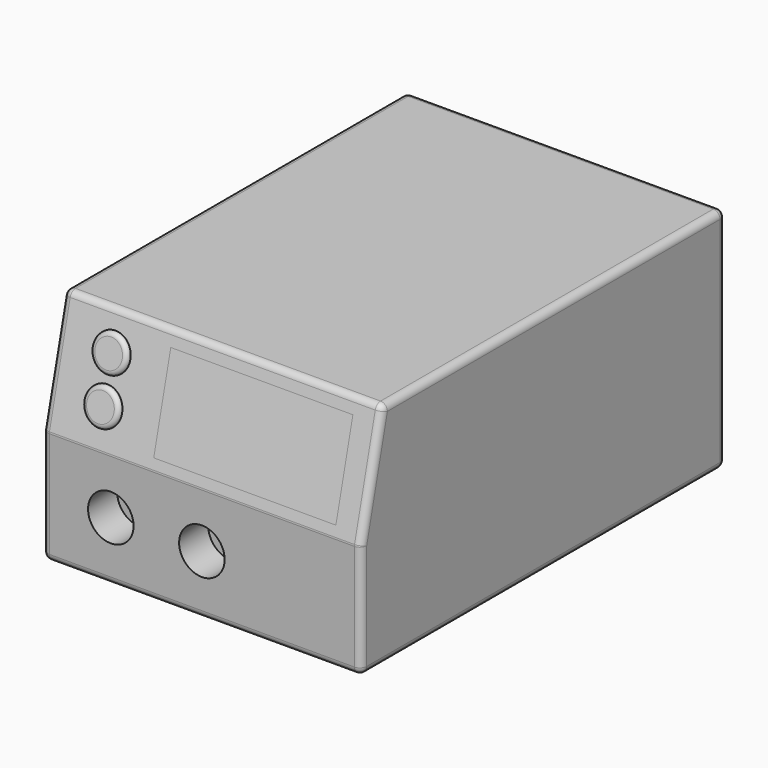
from build123d import *

# Parameters (mm, degrees)
F0_W      = 350
F0_H      = 500
F1_DEPTH  = 250
F3_DEPTH  = 350
F4_R      = 20
F5_DEPTH  = 5
F6_R      = 4.99999
F7_R      = 20
F8_DEPTH  = 5
F9_R      = 4.99999
F10_W     = 200
F10_H     = 100
F11_DEPTH = 5
F12_W     = 200
F12_H     = 100
F13_DEPTH = 5
F14_R     = 25
F15_DEPTH = 40
F16_R     = 7.5
F17_DEPTH = 60
F18_R     = 25
F19_DEPTH = 40
F20_R     = 7.5
F21_DEPTH = 60
F22_R     = 7.5
F23_R     = 12.5
F24_DEPTH = 30
F25_R     = 3
F26_DEPTH = 25
F27_W     = 55
F27_H     = 10
F28_DEPTH = 15


# Not quite as in the source:
# - a fillet or chamfer is up to 0.001 mm smaller than in the source, because OpenCascade refuses the exact size


with BuildPart() as f1:
    # F0 (on Top) → F1 (new body)
    with BuildSketch(Plane.XY):
        Rectangle(F0_W, F0_H)
    extrude(amount=F1_DEPTH)

    # F2 (on face) → F3 (cut)
    with BuildSketch(Plane.YZ.offset(175)):
        Polygon((-220, 250), (-250, 250), (-250, 125), align=None)
    extrude(amount=-F3_DEPTH, mode=Mode.SUBTRACT)

    # F10 (on face) → F11 (cut)
    with BuildSketch(Plane(origin=(0, -264.7503782148, 63.5400907716), x_dir=(1, 0, 0), z_dir=(0, -0.972387302, 0.2333729525))):
        with Locations((45, 124.7547759506)):
            Rectangle(F10_W, F10_H)
    extrude(amount=-F11_DEPTH, mode=Mode.SUBTRACT)

    # F14 (on face) → F15 (cut)
    with BuildSketch(Plane.XZ.offset(250)):
        with Locations((0, 65)):
            Circle(F14_R)
    extrude(amount=-F15_DEPTH, mode=Mode.SUBTRACT)

    # F16 (on face) → F17 (cut)
    with BuildSketch(Plane.XZ.offset(210)):
        with Locations((0, 65)):
            Circle(F16_R)
    extrude(amount=-F17_DEPTH, mode=Mode.SUBTRACT)

    # F18 (on face) → F19 (cut)
    with BuildSketch(Plane.XZ.offset(250)):
        with Locations((-100, 65)):
            Circle(F18_R)
    extrude(amount=-F19_DEPTH, mode=Mode.SUBTRACT)

    # F20 (on face) → F21 (cut)
    with BuildSketch(Plane.XZ.offset(210)):
        with Locations((-100, 65)):
            Circle(F20_R)
    extrude(amount=-F21_DEPTH, mode=Mode.SUBTRACT)

    # F22
    f22_edges = [f1.edges().sort_by_distance(p)[0] for p in [
        (175, -235, 187.5),
        (175, -250, 62.5),
        (0, -250, 125),
        (175, 15, 250),
        (175, 250, 125),
        (175, 0, 0),
        (0, -250, 0),
        (-175, -250, 62.5),
        (-175, -235, 187.5),
        (-175, 15, 250),
        (-175, 250, 125),
        (-175, 0, 0),
        (0, 250, 0),
        (0, 250, 250),
        (0, -220, 250),
    ]]
    fillet(f22_edges, radius=F22_R)

    # F23 (on face) → F24 (cut)
    with BuildSketch(Plane(origin=(0, 250, 0), x_dir=(-1, 0, 0), z_dir=(0, 1, 0))):
        with Locations((-132.5, 37.5)):
            Circle(F23_R)
    extrude(amount=-F24_DEPTH, mode=Mode.SUBTRACT)

    # F27 (on face) → F28 (cut)
    with BuildSketch(Plane(origin=(0, 250, 0), x_dir=(-1, 0, 0), z_dir=(0, 1, 0))):
        with Locations((-67.5, 37.5)):
            Rectangle(F27_W, F27_H)
    extrude(amount=-F28_DEPTH, mode=Mode.SUBTRACT)


with BuildPart() as f5:
    # F4 (on face) → F5 (new body)
    with BuildSketch(Plane(origin=(0, -264.7503782148, 63.5400907716), x_dir=(1, 0, 0), z_dir=(0, -0.972387302, 0.2333729525))):
        with Locations((-115, 151.7547759506)):
            Circle(F4_R)
    extrude(amount=F5_DEPTH)

    # F6 (radius 5 in the source; OpenCascade refuses exactly that, so slightly less here)
    f6_edges = [f5.edges().sort_by_distance(p)[0] for p in [
        (-135, -234.196855, 212.271373),
    ]]
    fillet(f6_edges, radius=F6_R)


with BuildPart() as f8:
    # F7 (on face) → F8 (new body)
    with BuildSketch(Plane(origin=(0, -264.7503782148, 63.5400907716), x_dir=(1, 0, 0), z_dir=(0, -0.972387302, 0.2333729525))):
        with Locations((-115, 103.2051746287)):
            Circle(F7_R)
    extrude(amount=F8_DEPTH)

    # F9 (radius 5 in the source; OpenCascade refuses exactly that, so slightly less here)
    f9_edges = [f8.edges().sort_by_distance(p)[0] for p in [
        (-135, -245.527018, 165.062357),
    ]]
    fillet(f9_edges, radius=F9_R)


with BuildPart() as f13:
    # F12 (on face) → F13 (new body)
    with BuildSketch(Plane(origin=(0, -264.7503782148, 63.5400907716), x_dir=(1, 0, 0), z_dir=(0, -0.972387302, 0.2333729525))):
        with Locations((45, 124.7547759506)):
            Rectangle(F12_W, F12_H)
    extrude(amount=-F13_DEPTH)


with BuildPart() as f26:
    # F25 (on face) → F26 (new body)
    with BuildSketch(Plane(origin=(0, 220, 0), x_dir=(-1, 0, 0), z_dir=(0, 1, 0))):
        with Locations((-132.5, 37.5)):
            Circle(F25_R)
    extrude(amount=F26_DEPTH)


solid = Compound([f1.part, f5.part, f8.part, f13.part, f26.part])
